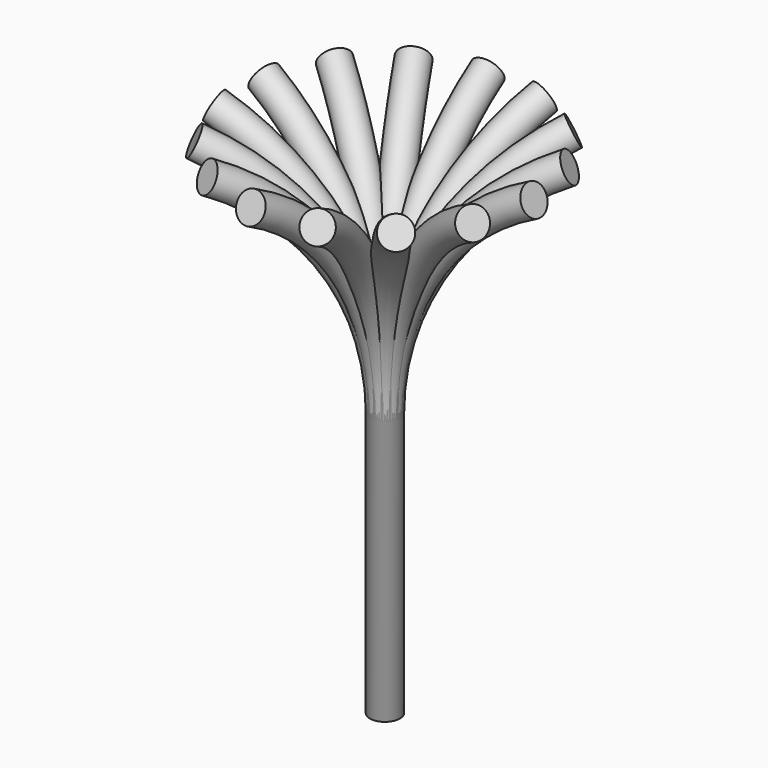
from build123d import *

# Parameters (mm, degrees)
F0_R     = 2.023840267
F3_COUNT = 15


with BuildPart() as f2:
    # F2: sweep along a path in F1
    with BuildLine(Plane.XZ) as f2_path:
        ThreePointArc((20.1003905386, 67.4798861146), (5.4453313374, 54.4625482788), (0, 35.6325134635))
        Line((0, 35.6325134635), (0, 0))
    # F0 (on Top) → F2 (sweep)
    with BuildSketch(Plane.XY):
        Circle(F0_R)
    sweep(path=f2_path.line)


with BuildPart() as f3_1:
    # F3: instance of F2
    add(f2.part.rotate(Axis((0, 0, 0), (0, 0, -1)), 1 * 360 / F3_COUNT))


with BuildPart() as f3_2:
    # F3: instance of F2
    add(f2.part.rotate(Axis((0, 0, 0), (0, 0, -1)), 2 * 360 / F3_COUNT))


with BuildPart() as f3_3:
    # F3: instance of F2
    add(f2.part.rotate(Axis((0, 0, 0), (0, 0, -1)), 3 * 360 / F3_COUNT))


with BuildPart() as f3_4:
    # F3: instance of F2
    add(f2.part.rotate(Axis((0, 0, 0), (0, 0, -1)), 4 * 360 / F3_COUNT))


with BuildPart() as f3_5:
    # F3: instance of F2
    add(f2.part.rotate(Axis((0, 0, 0), (0, 0, -1)), 5 * 360 / F3_COUNT))


with BuildPart() as f3_6:
    # F3: instance of F2
    add(f2.part.rotate(Axis((0, 0, 0), (0, 0, -1)), 6 * 360 / F3_COUNT))


with BuildPart() as f3_7:
    # F3: instance of F2
    add(f2.part.rotate(Axis((0, 0, 0), (0, 0, -1)), 7 * 360 / F3_COUNT))


with BuildPart() as f3_8:
    # F3: instance of F2
    add(f2.part.rotate(Axis((0, 0, 0), (0, 0, -1)), 8 * 360 / F3_COUNT))


with BuildPart() as f3_9:
    # F3: instance of F2
    add(f2.part.rotate(Axis((0, 0, 0), (0, 0, -1)), 9 * 360 / F3_COUNT))


with BuildPart() as f3_10:
    # F3: instance of F2
    add(f2.part.rotate(Axis((0, 0, 0), (0, 0, -1)), 10 * 360 / F3_COUNT))


with BuildPart() as f3_11:
    # F3: instance of F2
    add(f2.part.rotate(Axis((0, 0, 0), (0, 0, -1)), 11 * 360 / F3_COUNT))


with BuildPart() as f3_12:
    # F3: instance of F2
    add(f2.part.rotate(Axis((0, 0, 0), (0, 0, -1)), 12 * 360 / F3_COUNT))


with BuildPart() as f3_13:
    # F3: instance of F2
    add(f2.part.rotate(Axis((0, 0, 0), (0, 0, -1)), 13 * 360 / F3_COUNT))


with BuildPart() as f3_14:
    # F3: instance of F2
    add(f2.part.rotate(Axis((0, 0, 0), (0, 0, -1)), 14 * 360 / F3_COUNT))


solid = Compound([f2.part, f3_1.part, f3_2.part, f3_3.part, f3_4.part, f3_5.part, f3_6.part, f3_7.part, f3_8.part, f3_9.part, f3_10.part, f3_11.part, f3_12.part, f3_13.part, f3_14.part])
